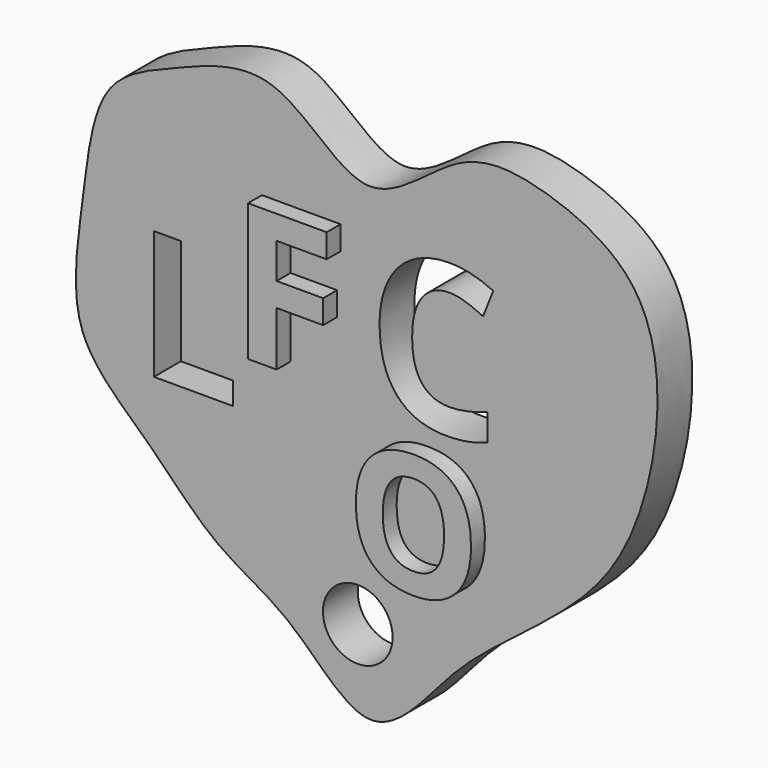
from build123d import *

# Parameters (mm, degrees)
F1_DEPTH     = 2.5
F2_TEXT_SIZE = 11.0513530672
F3_DEPTH     = 3.5
F4_TEXT_SIZE = 10.3402132582
F5_DEPTH     = 2.5
F6_TEXT_SIZE = 12.018223707
F7_DEPTH     = 2.5
F8_TEXT_SIZE = 9.73765402
F9_DEPTH     = 3.5
F10_R        = 2.0032715586
F11_DEPTH    = 2.5


# Not quite as in the source:
# - Text() gives the source's letters only with a copy of the font that has no kerning and outlines rounded to 1/6400 em; it was checked with that copy


with BuildPart() as f1:
    # F0 (on Front) → F1 (new body)
    with BuildSketch(Plane.XZ):
        with BuildLine():
            add(Edge.make_bspline(
                [(-33.5350890263, 35.1879246382), (-35.2998969271, 35.3038151175), (-38.647412148, 39.9920147643), (-44.5563525199, 37.5264684329), (-49.2569193195, 35.7618326799), (-49.8740577201, 29.0661064597), (-51.0285781057, 22.0781989326), (-46.1166637447, 18.2494682998), (-42.3890760352, 13.8563712046), (-37.7685276912, 12.05083321), (-33.3727077429, 6.2499647036), (-29.092887508, 11.7882768379), (-26.3418845014, 14.2133153902), (-21.1215392557, 17.9946935917), (-18.0760518253, 22.2662448543), (-16.4446055659, 29.0691572688), (-17.5182521705, 35.7743083488), (-23.5640346123, 38.5384168876), (-28.5007263966, 38.9298417213), (-31.827505737, 35.0757919547), (-33.5350890263, 35.1879246382)],
                knots=[0, 0, 0, 0, 0.0586734922, 0.1144066664, 0.1643154837, 0.2226933844, 0.2831951533, 0.3388678202, 0.3944595059, 0.4475314901, 0.5027336177, 0.5561976372, 0.6036940079, 0.6616288832, 0.7153195467, 0.7765782174, 0.8349561189, 0.8922345985, 0.9432290196, 1, 1, 1, 1], degree=3))
        make_face()
    extrude(amount=F1_DEPTH)

    # F2 (on Front) → F3 (join)
    with BuildSketch(Plane.XZ):
        with Locations((-40.6343713403, 24.8247496784)):
            Text('F', F2_TEXT_SIZE, font='Open Sans', font_style=FontStyle.BOLD, text_align=(TextAlign.LEFT, TextAlign.BOTTOM))
    extrude(amount=F3_DEPTH)

    # F4 (on Front) → F5 (cut, through all)
    with BuildSketch(Plane.XZ):
        with Locations((-46.7823855579, 21.4956048876)):
            Text('L', F4_TEXT_SIZE, font='Open Sans', font_style=FontStyle.BOLD, text_align=(TextAlign.LEFT, TextAlign.BOTTOM))
    extrude(amount=F5_DEPTH, mode=Mode.SUBTRACT)

    # F6 (on Front) → F7 (cut, through all)
    with BuildSketch(Plane.XZ):
        with Locations((-33.5734896362, 24.0957606584)):
            Text('C', F6_TEXT_SIZE, font='Open Sans', font_style=FontStyle.BOLD, text_align=(TextAlign.LEFT, TextAlign.BOTTOM))
    extrude(amount=F7_DEPTH, mode=Mode.SUBTRACT)

    # F8 (on Front) → F9 (join)
    with BuildSketch(Plane.XZ):
        with Locations((-34.0040847659, 16.0304149613)):
            Text('O', F8_TEXT_SIZE, font='Open Sans', font_style=FontStyle.BOLD, text_align=(TextAlign.LEFT, TextAlign.BOTTOM))
    extrude(amount=F9_DEPTH)

    # F10 (on Front) → F11 (cut, through all)
    with BuildSketch(Plane.XZ):
        with Locations((-34.1285169125, 12.7743463963)):
            Circle(F10_R)
    extrude(amount=F11_DEPTH, mode=Mode.SUBTRACT)


solid = f1.part
